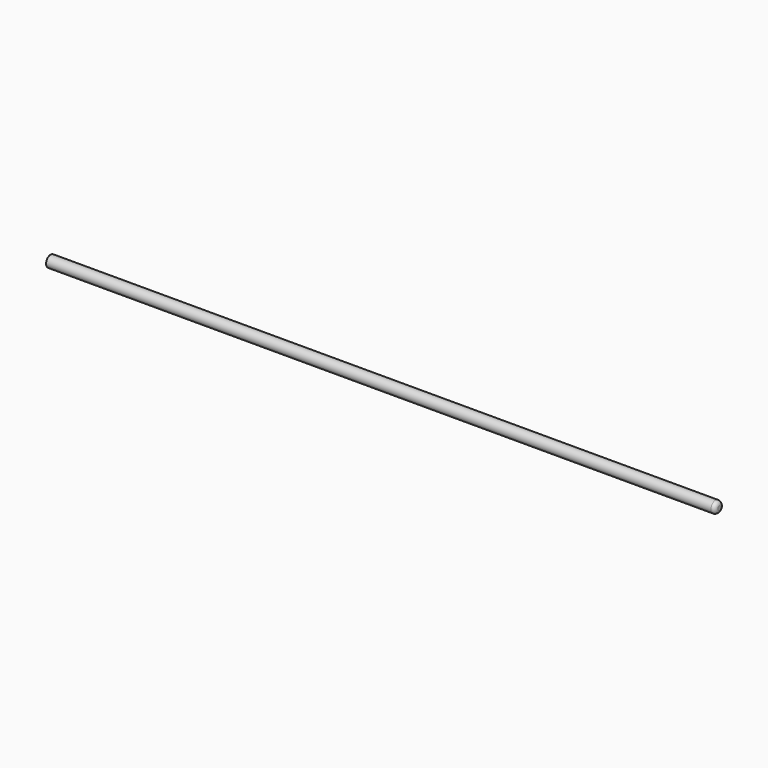
from build123d import *

# Parameters (mm, degrees)
F0_R     = 3
F0_R_2   = 2
F1_DEPTH = 350
F2_R     = 3.0183078128
F3_DEPTH = 2
F4_R     = 1.99999


# Not quite as in the source:
# - a fillet or chamfer is up to 0.001 mm smaller than in the source, because OpenCascade refuses the exact size


with BuildPart() as f1:
    # F0 (on Right) → F1 (new body)
    with BuildSketch(Plane.YZ):
        Circle(F0_R)
        Circle(F0_R_2, mode=Mode.SUBTRACT)
    extrude(amount=F1_DEPTH)

    # F2 (on face) → F3 (join)
    with BuildSketch(Plane.YZ.offset(350)):
        Circle(F2_R)
    extrude(amount=F3_DEPTH)

    # F4 (radius 2 in the source; OpenCascade refuses exactly that, so slightly less here)
    f4_edges = [f1.edges().sort_by_distance(p)[0] for p in [
        (352, -3.018308, 0),
    ]]
    fillet(f4_edges, radius=F4_R)


solid = f1.part
